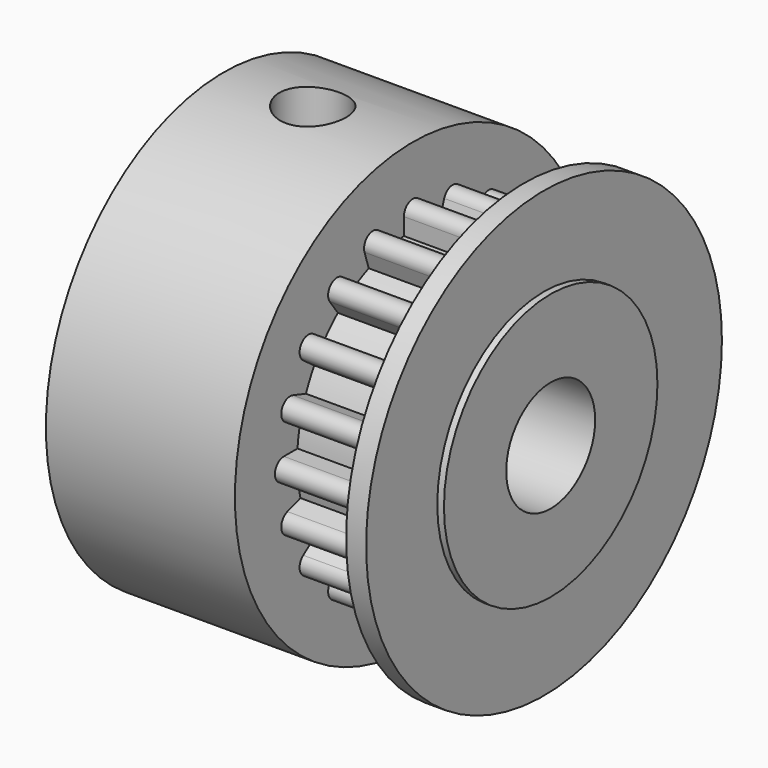
from build123d import *

# Parameters (mm, degrees)
F0_R            = 10
F1_DEPTH        = 8.5
F3_DEPTH        = 5
F3_COPIES_COUNT = 20
F5_R            = 10
F6_DEPTH        = 0.9
F7_R            = 6
F8_DEPTH        = 0.3
F9_R            = 2.5
F10_DEPTH       = 14.7
F11_R           = 1.5
F12_REACH       = 14.2436406871


# Not quite as in the source:
# - a pattern or mirror of a feature is missing from the dataset's text; its kind, count and spacing are read off the source's solid


with BuildPart() as f1:
    # F0 (on Right) → F1 (new body)
    with BuildSketch(Plane.YZ):
        Circle(F0_R)
    extrude(amount=F1_DEPTH)

    # F2 (on face) → F3 (join)
    with BuildSketch(Plane.YZ.offset(8.5)):
        with BuildLine():
            Line((0.5, 6.4807406984), (0.5, 7.25))
            ThreePointArc((0.5, 7.25), (0, 7.75), (-0.5, 7.25))
            Line((-0.5, 7.25), (-0.5, 6.4807406984))
            ThreePointArc((-0.5, 6.4807406984), (0, -6.5), (0.5, 6.4807406984))
        make_face()
    f3 = extrude(amount=F3_DEPTH)

    # F3_copies: F3 ×20 about axis
    f3_copies_axis = Axis((0, 0, 0), (1, 0, 0))
    for i in range(1, F3_COPIES_COUNT):
        add(f3.rotate(f3_copies_axis, i * 360 / F3_COPIES_COUNT))

    # F5 (on face) → F6 (join)
    with BuildSketch(Plane.YZ.offset(13.5)):
        Circle(F5_R)
    extrude(amount=F6_DEPTH)

    # F7 (on face) → F8 (join)
    with BuildSketch(Plane.YZ.offset(14.4)):
        Circle(F7_R)
    extrude(amount=F8_DEPTH)

    # F9 (on face) → F10 (cut, through all)
    with BuildSketch(Plane.YZ.offset(14.7)):
        Circle(F9_R)
    extrude(amount=-F10_DEPTH, mode=Mode.SUBTRACT)

    f12_end = f1.faces().sort_by_distance((4.25, -10, 0))[0]
    # F11 (on Top) → F12 (cut, up to a face of the model that its end follows)
    with BuildSketch(Plane.XY):
        with Locations((4, 0)):
            Circle(F11_R)
    f12_long = extrude(amount=F12_REACH, mode=Mode.PRIVATE)
    add(split(f12_long, bisect_by=f12_end, keep=Keep.BOTTOM, mode=Mode.PRIVATE), mode=Mode.SUBTRACT)


solid = f1.part
